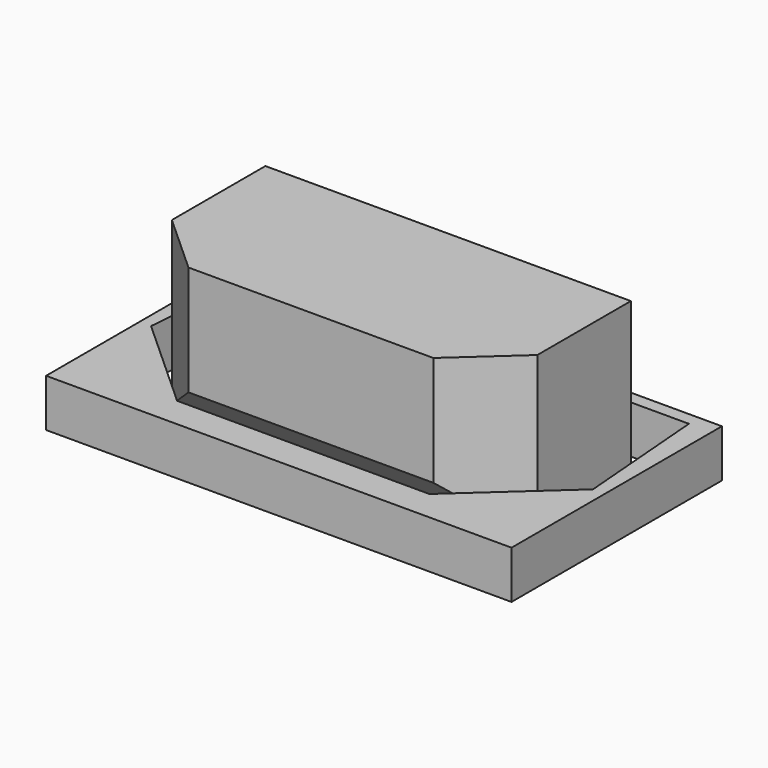
from build123d import *

# Parameters (mm, degrees)
F0_W     = 974.2202758789
F0_H     = 550.4953376949
F1_DEPTH = 100
F3_DEPTH = 340
F5_DEPTH = 950.088428093


with BuildPart() as f1:
    # F0 (on Top) → F1 (new body)
    with BuildSketch(Plane.XY):
        with Locations((462.9772901535, 245.6912044436)):
            Rectangle(F0_W, F0_H)
        Polygon((237.0983631819, 0), (0, 0), (0, 35), (0, 214.90548196), (0, 312), (0, 379), (0, 494), (22.5, 494), (462.5, 494), (902.5, 494), (925, 494), (925, 379), (925, 312), (925, 214.90548196), (925, 35), (925, 0), (687.9016368181, 0), (462.5, 0), align=None, mode=Mode.SUBTRACT)
        Polygon((0, 494), (0, 379), (13.2289472464, 379), (22.5, 494), align=None)
        Polygon((902.5, 494), (911.7710527536, 379), (925, 379), (925, 494), align=None)
        Polygon((925, 214.90548196), (726.5160203865, 35), (925, 35), align=None)
        Polygon((726.5160203865, 35), (687.9016368181, 0), (925, 0), (925, 35), align=None)
        Polygon((0, 35), (0, 0), (237.0983631819, 0), (198.4839796135, 35), align=None)
        Polygon((0, 214.90548196), (0, 35), (198.4839796135, 35), align=None)
        Polygon((0, 379), (0, 312), (7.8275512942, 312), (13.2289472464, 379), align=None)
        Polygon((0, 312), (0, 214.90548196), (7.8275512942, 312), align=None)
        Polygon((917.1724487058, 312), (925, 214.90548196), (925, 312), align=None)
        Polygon((911.7710527536, 379), (917.1724487058, 312), (925, 312), (925, 379), align=None)
        Polygon((462.5, 35), (462.5, 0), (687.9016368181, 0), (726.5160203865, 35), align=None)
        Polygon((198.4839796135, 35), (237.0983631819, 0), (462.5, 0), (462.5, 35), align=None)
    extrude(amount=F1_DEPTH)


with BuildPart() as f3:
    # F2 (on Top) → F3 (new body)
    with BuildSketch(Plane.XY):
        Polygon((845, 414), (80, 414), (80, 169.3866584137), (206.1991515171, 55), (718.8008484829, 55), (845, 169.3866584137), align=None)
    extrude(amount=F3_DEPTH)

    # F4 (on Right) → F5 (cut, through all)
    with BuildSketch(Plane.YZ):
        Polygon((55, 0), (169.3866584137, 0), (55, 110), align=None)
    extrude(amount=F5_DEPTH, mode=Mode.SUBTRACT)


solid = Compound([f1.part, f3.part])
